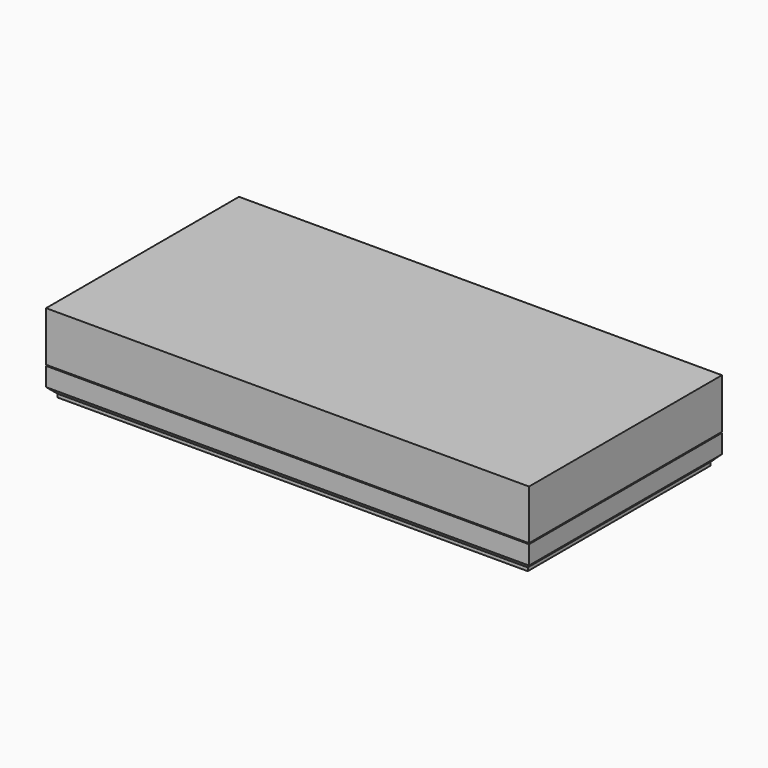
from build123d import *

# Parameters (mm, degrees)
F4_W          = 145.8
F4_H          = 72.8
F5_DEPTH      = 1
F6_W          = 145.8
F6_H          = 72.8
F6_W_2        = 138.8
F6_H_2        = 65.8
F7_DEPTH      = 10.85
F8_W          = 2
F8_H          = 10.85
F9_DEPTH      = 65.8
F12_W         = 145.8
F12_H         = 72.8
F12_W_2       = 142
F12_H_2       = 69
F13_DEPTH     = 3.3
F14_W         = 145.8
F14_H         = 72.8
F14_W_2       = 142
F14_H_2       = 69
F15_DEPTH     = 3
F16_T4_DEPTH  = 142
F16_T9_DEPTH  = 69
F16_T14_DEPTH = 142
F16_T19_DEPTH = 69
F16_T25_DEPTH = 147.1433659759
F16_T31_DEPTH = 74.1433659759
F16_T40_DEPTH = 147.1433659759
F16_T46_DEPTH = 74.1433659759
F16_T55_DEPTH = 147.1433659759
F16_T61_DEPTH = 74.1433659759
F16_T70_DEPTH = 74.1433659759
F16_T76_DEPTH = 147.1433659759
F17_W         = 145.8
F17_H         = 72.8
F17_W_2       = 142.6
F17_H_2       = 69.6
F18_DEPTH     = 3.2


# Not quite as in the source:
# - a fillet or chamfer that OpenCascade refuses, or shapes differently, is made with other operations: its cross-section is extruded or revolved along the edge and cut away or added


with BuildPart() as f5:
    # F4 (on Top) → F5 (new body)
    with BuildSketch(Plane.XY):
        Rectangle(F4_W, F4_H)
    extrude(amount=F5_DEPTH)

    # F6 (on face) → F7 (join)
    with BuildSketch(Plane.XY.offset(1)):
        Rectangle(F6_W, F6_H)
        Rectangle(F6_W_2, F6_H_2, mode=Mode.SUBTRACT)
    extrude(amount=F7_DEPTH)

    # F8 (on face) → F9 (join, through all)
    with BuildSketch(Plane.XZ.offset(-32.9)):
        with Locations((-35.2, 6.425)):
            Rectangle(F8_W, F8_H)
        with Locations((16.3, 6.425)):
            Rectangle(F8_W, F8_H)
        with Locations((35.2, 6.425)):
            Rectangle(F8_W, F8_H)
    extrude(amount=F9_DEPTH)


with BuildPart() as f11_1:
    # F11: instance of F5
    add(f5.part.mirror(Plane(origin=(1.1434328358, 0, 11.95), x_dir=(1, 0, 0), z_dir=(0, 0, 1))))

    # F17 (on face) → F18 (join)
    with BuildSketch(Plane(origin=(0, 0, 12.05), x_dir=(1, 0, 0), z_dir=(0, 0, -1))):
        Rectangle(F17_W, F17_H)
        Rectangle(F17_W_2, F17_H_2, mode=Mode.SUBTRACT)
    extrude(amount=F18_DEPTH)


with BuildPart() as f5_1:
    add(f5.part)

    # F12 (on face) → F13 (cut)
    with BuildSketch(Plane.XY.offset(11.85)):
        Rectangle(F12_W, F12_H)
        Rectangle(F12_W_2, F12_H_2, mode=Mode.SUBTRACT)
    extrude(amount=-F13_DEPTH, mode=Mode.SUBTRACT)

    # F14 (on face) → F15 (cut)
    with BuildSketch(Plane(origin=(0, 0, 0), x_dir=(1, 0, 0), z_dir=(0, 0, -1))):
        Rectangle(F14_W, F14_H)
        Rectangle(F14_W_2, F14_H_2, mode=Mode.SUBTRACT)
    extrude(amount=-F15_DEPTH, mode=Mode.SUBTRACT)

    # F16: chamfer of 2 on 4 edges, made by hand


with BuildPart() as f16_tool2:
    # F16_s3 → F16_t4 (new body)
    with BuildSketch(Plane.YZ.offset(-71)):
        Polygon((-36.5, 3), (-34.5, 1), (-34.5, 3), align=None)
    extrude(amount=F16_T4_DEPTH)

    split(bisect_by=Plane.XZ.offset(36.4), keep=Keep.BOTTOM)


with BuildPart() as f5_2:
    add(f5_1.part)

    # F16_t1: union F16_tool2
    add(f16_tool2.part)


with BuildPart() as f16_tool7:
    # F16_s8 → F16_t9 (new body)
    with BuildSketch(Plane.XZ.offset(-34.5)):
        Polygon((-73, 3), (-71, 1), (-71, 3), align=None)
    extrude(amount=F16_T9_DEPTH)

    split(bisect_by=Plane.YZ.offset(-72.9), keep=Keep.TOP)


with BuildPart() as f5_3:
    add(f5_2.part)

    # F16_t6: union F16_tool7
    add(f16_tool7.part)


with BuildPart() as f16_tool12:
    # F16_s13 → F16_t14 (new body)
    with BuildSketch(Plane.YZ.offset(71)):
        Polygon((36.5, 3), (34.5, 1), (34.5, 3), align=None)
    extrude(amount=-F16_T14_DEPTH)

    split(bisect_by=Plane.XZ.offset(-36.4), keep=Keep.TOP)


with BuildPart() as f5_4:
    add(f5_3.part)

    # F16_t11: union F16_tool12
    add(f16_tool12.part)


with BuildPart() as f16_tool17:
    # F16_s18 → F16_t19 (new body)
    with BuildSketch(Plane.XZ.offset(34.5)):
        Polygon((73, 3), (71, 1), (71, 3), align=None)
    extrude(amount=-F16_T19_DEPTH)

    split(bisect_by=Plane.YZ.offset(72.9), keep=Keep.BOTTOM)


with BuildPart() as f5_5:
    add(f5_4.part)

    # F16_t16: union F16_tool17
    add(f16_tool17.part)


with BuildPart() as f16_tool23:
    # F16_s24 → F16_t25 (new body)
    with BuildSketch(Plane.YZ.offset(-76.1433659759)):
        Polygon((-36.5, 3), (-34.5, 1), (-34.5, 3), align=None)
    extrude(amount=F16_T25_DEPTH)

    split(bisect_by=Plane.XZ.offset(36.4), keep=Keep.BOTTOM)

    split(bisect_by=Plane.YZ.offset(-72.9), keep=Keep.TOP)

    split(bisect_by=Plane.YZ.offset(-71), keep=Keep.BOTTOM)


with BuildPart() as f16_tool29:
    # F16_s30 → F16_t31 (new body)
    with BuildSketch(Plane.XZ.offset(-34.5)):
        Polygon((-73, 3), (-71, 1), (-71, 3), align=None)
    extrude(amount=F16_T31_DEPTH)

    split(bisect_by=Plane.XZ.offset(36.4), keep=Keep.BOTTOM)

    split(bisect_by=Plane.YZ.offset(-72.9), keep=Keep.TOP)

    split(bisect_by=Plane.XZ.offset(34.5), keep=Keep.TOP)


with BuildPart() as f16_tool23_1:
    add(f16_tool23.part)

    # F16_t35: intersect F16_tool29
    add(f16_tool29.part, mode=Mode.INTERSECT)


with BuildPart() as f5_6:
    add(f5_5.part)

    # F16_t21: union F16_tool23
    add(f16_tool23_1.part)


with BuildPart() as f16_tool38:
    # F16_s39 → F16_t40 (new body)
    with BuildSketch(Plane.YZ.offset(-71)):
        Polygon((-36.5, 3), (-34.5, 1), (-34.5, 3), align=None)
    extrude(amount=F16_T40_DEPTH)

    split(bisect_by=Plane.XZ.offset(36.4), keep=Keep.BOTTOM)

    split(bisect_by=Plane.YZ.offset(72.9), keep=Keep.BOTTOM)

    split(bisect_by=Plane.YZ.offset(71), keep=Keep.TOP)


with BuildPart() as f16_tool44:
    # F16_s45 → F16_t46 (new body)
    with BuildSketch(Plane.XZ.offset(39.6433659759)):
        Polygon((73, 3), (71, 1), (71, 3), align=None)
    extrude(amount=-F16_T46_DEPTH)

    split(bisect_by=Plane.XZ.offset(36.4), keep=Keep.BOTTOM)

    split(bisect_by=Plane.YZ.offset(72.9), keep=Keep.BOTTOM)

    split(bisect_by=Plane.XZ.offset(34.5), keep=Keep.TOP)


with BuildPart() as f16_tool38_1:
    add(f16_tool38.part)

    # F16_t50: intersect F16_tool44
    add(f16_tool44.part, mode=Mode.INTERSECT)


with BuildPart() as f5_7:
    add(f5_6.part)

    # F16_t36: union F16_tool38
    add(f16_tool38_1.part)


with BuildPart() as f16_tool53:
    # F16_s54 → F16_t55 (new body)
    with BuildSketch(Plane.YZ.offset(71)):
        Polygon((36.5, 3), (34.5, 1), (34.5, 3), align=None)
    extrude(amount=-F16_T55_DEPTH)

    split(bisect_by=Plane.YZ.offset(-72.9), keep=Keep.TOP)

    split(bisect_by=Plane.XZ.offset(-36.4), keep=Keep.TOP)

    split(bisect_by=Plane.YZ.offset(-71), keep=Keep.BOTTOM)


with BuildPart() as f16_tool59:
    # F16_s60 → F16_t61 (new body)
    with BuildSketch(Plane.XZ.offset(-39.6433659759)):
        Polygon((-73, 3), (-71, 1), (-71, 3), align=None)
    extrude(amount=F16_T61_DEPTH)

    split(bisect_by=Plane.YZ.offset(-72.9), keep=Keep.TOP)

    split(bisect_by=Plane.XZ.offset(-36.4), keep=Keep.TOP)

    split(bisect_by=Plane.XZ.offset(-34.5), keep=Keep.BOTTOM)


with BuildPart() as f16_tool53_1:
    add(f16_tool53.part)

    # F16_t65: intersect F16_tool59
    add(f16_tool59.part, mode=Mode.INTERSECT)


with BuildPart() as f5_8:
    add(f5_7.part)

    # F16_t51: union F16_tool53
    add(f16_tool53_1.part)


with BuildPart() as f16_tool68:
    # F16_s69 → F16_t70 (new body)
    with BuildSketch(Plane.XZ.offset(34.5)):
        Polygon((73, 3), (71, 1), (71, 3), align=None)
    extrude(amount=-F16_T70_DEPTH)

    split(bisect_by=Plane.YZ.offset(72.9), keep=Keep.BOTTOM)

    split(bisect_by=Plane.XZ.offset(-36.4), keep=Keep.TOP)

    split(bisect_by=Plane.XZ.offset(-34.5), keep=Keep.BOTTOM)


with BuildPart() as f16_tool74:
    # F16_s75 → F16_t76 (new body)
    with BuildSketch(Plane.YZ.offset(76.1433659759)):
        Polygon((36.5, 3), (34.5, 1), (34.5, 3), align=None)
    extrude(amount=-F16_T76_DEPTH)

    split(bisect_by=Plane.YZ.offset(72.9), keep=Keep.BOTTOM)

    split(bisect_by=Plane.XZ.offset(-36.4), keep=Keep.TOP)

    split(bisect_by=Plane.YZ.offset(71), keep=Keep.TOP)


with BuildPart() as f16_tool68_1:
    add(f16_tool68.part)

    # F16_t80: intersect F16_tool74
    add(f16_tool74.part, mode=Mode.INTERSECT)


with BuildPart() as f5_9:
    add(f5_8.part)

    # F16_t66: union F16_tool68
    add(f16_tool68_1.part)


solid = Compound([f11_1.part, f5_9.part])
